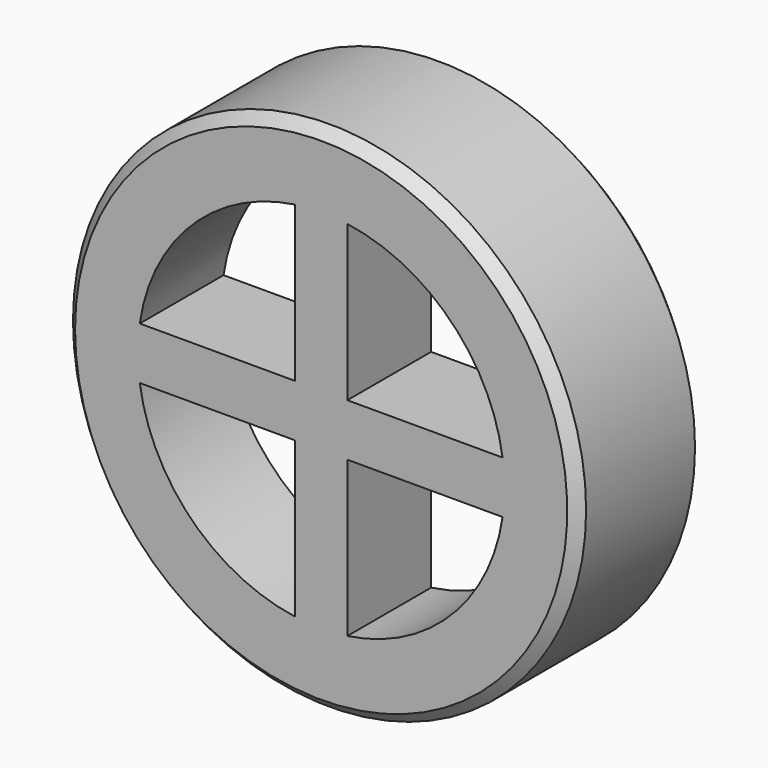
from build123d import *

# Parameters (mm, degrees)
F3_DEPTH = 25
F4_SIZE  = 0.99999


# Not quite as in the source:
# - a fillet or chamfer is up to 0.001 mm smaller than in the source, because OpenCascade refuses the exact size


with BuildPart() as f1:
    # F0 (on Top) → F1 (revolve)
    with BuildSketch(Plane.XY):
        Polygon((-24.5, 15), (-24.5, 0), (0, 0), (0, 10), (-21, 10), (-21, 5), (-23.5, 5), (-23.5, 15), align=None)
    revolve(axis=Axis((0, 1.7348257825, 0), (0, 1, 0)))

    # F2 (on face) → F3 (cut)
    with BuildSketch(Plane(origin=(0, 10, 0), x_dir=(-1, 0, 0), z_dir=(0, 1, 0))):
        with BuildLine():
            Line((-2.5, -2.5), (-17.3205080757, -2.5))
            ThreePointArc((-17.3205080757, -2.5), (-12.3743686708, -12.3743686708), (-2.5, -17.3205080757))
            Line((-2.5, -17.3205080757), (-2.5, -2.5))
        make_face()
        with BuildLine():
            ThreePointArc((17.3205080757, 2.5), (12.3743686708, 12.3743686708), (2.5, 17.3205080757))
            Line((2.5, 17.3205080757), (2.5, 2.5))
            Line((2.5, 2.5), (17.3205080757, 2.5))
        make_face()
        with BuildLine():
            Line((-2.5, 2.5), (-2.5, 17.3205080757))
            ThreePointArc((-2.5, 17.3205080757), (-12.3743686708, 12.3743686708), (-17.3205080757, 2.5))
            Line((-17.3205080757, 2.5), (-2.5, 2.5))
        make_face()
        with BuildLine():
            Line((17.3205080757, -2.5), (2.5, -2.5))
            Line((2.5, -2.5), (2.5, -17.3205080757))
            ThreePointArc((2.5, -17.3205080757), (12.3743686708, -12.3743686708), (17.3205080757, -2.5))
        make_face()
    extrude(amount=-F3_DEPTH, mode=Mode.SUBTRACT)

    # F4 (size 1 in the source; OpenCascade refuses exactly that, so slightly less here)
    f4_edges = [f1.edges().sort_by_distance(p)[0] for p in [
        (24.5, 0, 0),
        (24.5, 15, 0),
        (21, 10, 0),
    ]]
    chamfer(f4_edges, length=F4_SIZE)


solid = f1.part
